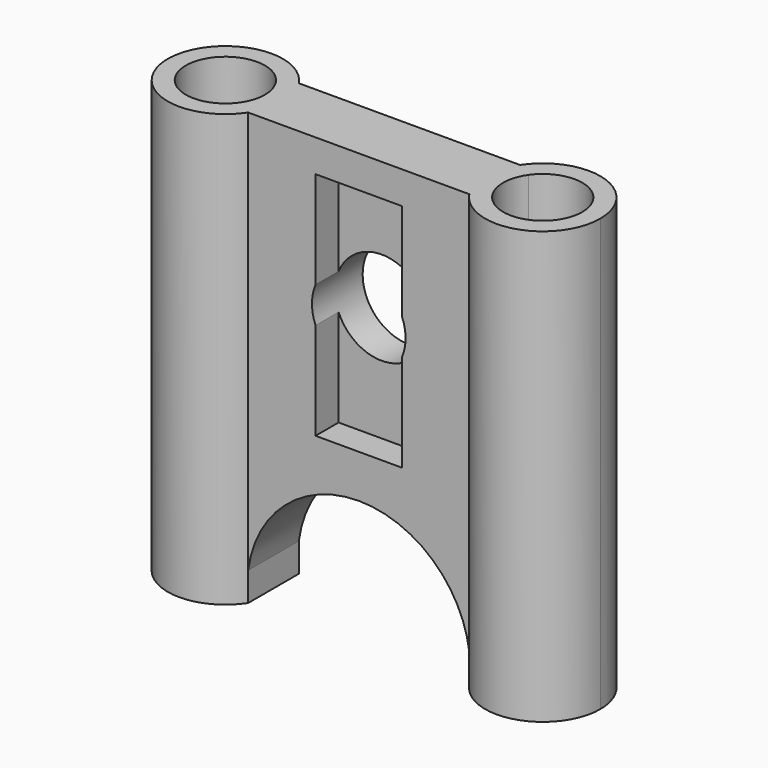
from build123d import *

# Parameters (mm, degrees)
F1_DEPTH = 30
F3_DEPTH = 4.4
F4_DEPTH = 2
F5_DEPTH = 2.4
F7_DEPTH = 4.4


with BuildPart() as f1:
    # F0 (on Top) → F1 (new body)
    with BuildSketch(Plane.XY):
        with BuildLine():
            Line((7.8582108495, 2.1976148234), (7.8582108495, 1.5812813318))
            Line((7.8582108495, 1.5812813318), (7.8582108495, -2.1976148234))
            ThreePointArc((7.8582108495, -2.1976148234), (12.3474105352, -3.8320303136), (15.2004390117, 0))
            ThreePointArc((15.2004390117, 0), (12.3474105352, 3.8320303136), (7.8582108495, 2.1976148234))
        make_face()
        with BuildLine():
            ThreePointArc((8.9505391584, 1.5812813318), (12.0296782424, 2.6219958616), (13.9504390117, 0))
            ThreePointArc((13.9504390117, 0), (10.3711997809, -2.6219958616), (8.9505391584, 1.5812813318))
        make_face(mode=Mode.SUBTRACT)
        with BuildLine():
            Line((7.8582108495, -2.1976148234), (7.8582108495, 1.5812813318))
            Line((7.8582108495, 1.5812813318), (7.5262657237, 1.5812813318))
            ThreePointArc((7.5262657237, 1.5812813318), (7.2157826444, -0.3500194778), (7.8582108495, -2.1976148234))
        make_face()
        with BuildLine():
            Line((7.5262657237, 1.5812813318), (7.8582108495, 1.5812813318))
            Line((7.8582108495, 1.5812813318), (7.8582108495, 2.1976148234))
            ThreePointArc((7.8582108495, 2.1976148234), (7.6787293316, 1.8967237357), (7.5262657237, 1.5812813318))
        make_face()
        with BuildLine():
            ThreePointArc((7.8582108495, -2.1976148234), (7.2157826444, -0.3500194778), (7.5262657237, 1.5812813318))
            Line((7.5262657237, 1.5812813318), (-7.1725568309, 1.5812813318))
            ThreePointArc((-7.1725568309, 1.5812813318), (-6.9290335283, 0.8072505337), (-6.8467301189, 0))
            ThreePointArc((-6.8467301189, 0), (-7.0146998053, -1.1469715235), (-7.5045019567, -2.1976148234))
            Line((-7.5045019567, -2.1976148234), (7.8582108495, -2.1976148234))
        make_face()
        with BuildLine():
            Line((-7.1725568309, 1.5812813318), (7.5262657237, 1.5812813318))
            ThreePointArc((7.5262657237, 1.5812813318), (7.6787293316, 1.8967237357), (7.8582108495, 2.1976148234))
            Line((7.8582108495, 2.1976148234), (7.8582108495, 2.2023851766))
            Line((7.8582108495, 2.2023851766), (-7.5076434872, 2.2023851766))
            ThreePointArc((-7.5076434872, 2.2023851766), (-7.3263755669, 1.8992376967), (-7.1725568309, 1.5812813318))
        make_face()
        with BuildLine():
            ThreePointArc((-6.8467301189, 0), (-6.9290335283, 0.8072505337), (-7.1725568309, 1.5812813318))
            Line((-7.1725568309, 1.5812813318), (-7.5076434872, 1.5812813318))
            Line((-7.5076434872, 1.5812813318), (-7.5076434872, -2.1976148234))
            Line((-7.5076434872, -2.1976148234), (-7.5045019567, -2.1976148234))
            ThreePointArc((-7.5045019567, -2.1976148234), (-7.0146998053, -1.1469715235), (-6.8467301189, 0))
        make_face()
        with BuildLine():
            Line((-7.5076434872, 1.5812813318), (-7.1725568309, 1.5812813318))
            ThreePointArc((-7.1725568309, 1.5812813318), (-7.3263755669, 1.8992376967), (-7.5076434872, 2.2023851766))
            Line((-7.5076434872, 2.2023851766), (-7.5076434872, 1.5812813318))
        make_face()
        with BuildLine():
            ThreePointArc((-7.5076434872, 2.2023851766), (-14.8467290993, -0.0028559361), (-7.5045019567, -2.1976148234))
            Line((-7.5045019567, -2.1976148234), (-7.5076434872, -2.1976148234))
            Line((-7.5076434872, -2.1976148234), (-7.5076434872, 1.5812813318))
            Line((-7.5076434872, 1.5812813318), (-7.5076434872, 2.2023851766))
        make_face()
        with BuildLine():
            ThreePointArc((-8.0967301189, 0), (-13.4687259805, -0.8292392307), (-8.5968302656, 1.5812813318))
            ThreePointArc((-8.5968302656, 1.5812813318), (-8.2247342573, 0.8292392307), (-8.0967301189, 0))
        make_face(mode=Mode.SUBTRACT)
    extrude(amount=F1_DEPTH)

    # F2 (on face) → F3 (cut, through all)
    with BuildSketch(Plane.XZ.offset(2.1976148234)):
        with BuildLine():
            Line((3.1768544464, 18.5), (3.1768544464, 21))
            ThreePointArc((3.1768544464, 21), (0.1768544464, 23), (-2.8231455536, 21))
            Line((-2.8231455536, 21), (-2.8231455536, 18.5))
            ThreePointArc((-2.8231455536, 18.5), (0.1768544464, 16.5), (3.1768544464, 18.5))
        make_face()
    extrude(amount=-F3_DEPTH, mode=Mode.SUBTRACT)

    # F2 (on face) → F4 (cut)
    with BuildSketch(Plane.XZ.offset(2.1976148234)):
        with BuildLine():
            ThreePointArc((3.1768544464, 18.5), (3.3637416424, 19.1126225608), (3.4268544464, 19.75))
            ThreePointArc((3.4268544464, 19.75), (3.3637416424, 20.3873774392), (3.1768544464, 21))
            Line((3.1768544464, 21), (3.1768544464, 18.5))
        make_face()
        with BuildLine():
            Line((3.1768544464, 18.5), (3.1768544464, 21))
            ThreePointArc((3.1768544464, 21), (0.1768544464, 23), (-2.8231455536, 21))
            Line((-2.8231455536, 21), (-2.8231455536, 18.5))
            ThreePointArc((-2.8231455536, 18.5), (0.1768544464, 16.5), (3.1768544464, 18.5))
        make_face()
        with BuildLine():
            ThreePointArc((-2.8231455536, 21), (0.1768544464, 23), (3.1768544464, 21))
            Line((3.1768544464, 21), (3.1768544464, 27.75))
            Line((3.1768544464, 27.75), (-2.8231455536, 27.75))
            Line((-2.8231455536, 27.75), (-2.8231455536, 21))
        make_face()
        with BuildLine():
            Line((3.1768544464, 11.75), (3.1768544464, 18.5))
            ThreePointArc((3.1768544464, 18.5), (0.1768544464, 16.5), (-2.8231455536, 18.5))
            Line((-2.8231455536, 18.5), (-2.8231455536, 11.75))
            Line((-2.8231455536, 11.75), (3.1768544464, 11.75))
        make_face()
        with BuildLine():
            Line((-2.8231455536, 18.5), (-2.8231455536, 21))
            ThreePointArc((-2.8231455536, 21), (-3.0731455536, 19.75), (-2.8231455536, 18.5))
        make_face()
    extrude(amount=-F4_DEPTH, mode=Mode.SUBTRACT)

    # F5 (cut, through all): faces of the model
    f5_faces = [f1.faces().sort_by_distance(p)[0] for p in [
        (-2.9234827298, -0.1976148234, 19.75),
        (3.2771916226, -0.1976148234, 19.75),
    ]]
    extrude(f5_faces, amount=-F5_DEPTH, mode=Mode.SUBTRACT)

    # F6 (on face) → F7 (cut, through all)
    with BuildSketch(Plane.XZ.offset(2.1976148234)):
        with BuildLine():
            Line((-7.5045019567, 0), (7.8582108495, 0))
            Line((7.8582108495, 0), (7.8582108495, 2.0067730067))
            ThreePointArc((7.8582108495, 2.0067730067), (0.1768544464, 8.75), (-7.5045019567, 2.0067730067))
            Line((-7.5045019567, 2.0067730067), (-7.5045019567, 0))
        make_face()
    extrude(amount=-F7_DEPTH, mode=Mode.SUBTRACT)


solid = f1.part
